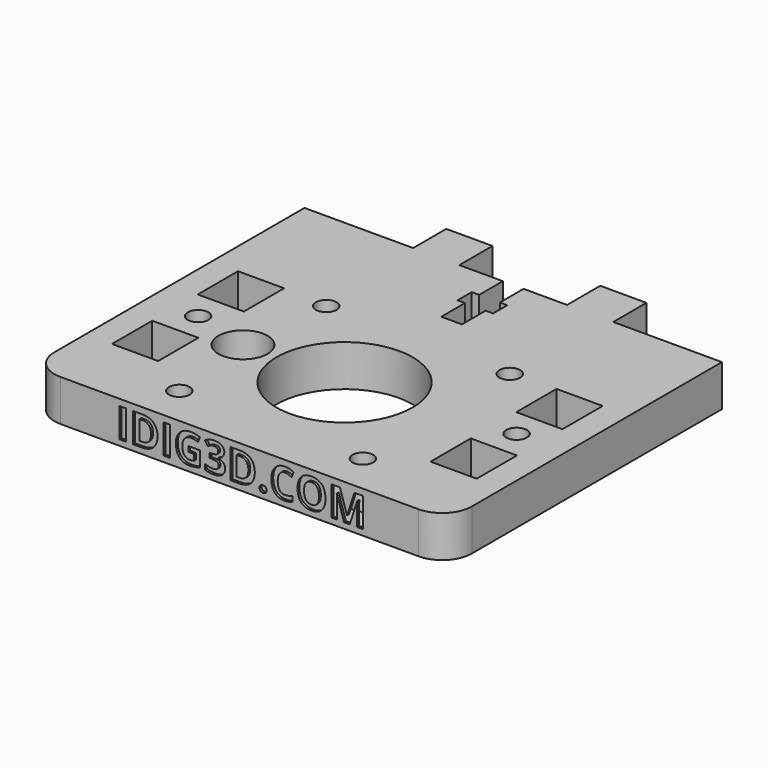
from build123d import *

# Parameters (mm, degrees)
F0_W         = 7.8
F0_H         = 7
F0_H_2       = 8.5
F0_R         = 1.75
F0_R_2       = 4.15
F0_R_3       = 11.5
F1_DEPTH     = 7
F2_TEXT_SIZE = 6.9444444444
F3_DEPTH     = 0.4


# Not quite as in the source:
# - Text() gives the source's letters only with a copy of the font that has no kerning and outlines rounded to 1/6400 em; it was checked with that copy


with BuildPart() as f1:
    # F0 (on Top) → F1 (new body)
    with BuildSketch(Plane.XY):
        with Locations((-13, 32.4)):
            Rectangle(F0_W, F0_H)
        with Locations((13, 32.4)):
            Rectangle(F0_W, F0_H)
        with BuildLine():
            Line((-16.9, 28.9), (-35.25, 28.9))
            Line((-35.25, 28.9), (-35.25, -23.9))
            ThreePointArc((-35.25, -23.9), (-33.7855339059, -27.4355339059), (-30.25, -28.9))
            Line((-30.25, -28.9), (30.25, -28.9))
            ThreePointArc((30.25, -28.9), (33.7855339059, -27.4355339059), (35.25, -23.9))
            Line((35.25, -23.9), (35.25, 28.9))
            Line((35.25, 28.9), (16.9, 28.9))
            Line((16.9, 28.9), (9.1, 28.9))
            Line((9.1, 28.9), (1.75, 28.9))
            Line((1.75, 28.9), (1.75, 23.9))
            Line((1.75, 23.9), (3, 23.9))
            Line((3, 23.9), (3, 20.9))
            Line((3, 20.9), (1.75, 20.9))
            Line((1.75, 20.9), (1.75, 15.9))
            Line((1.75, 15.9), (-1.75, 15.9))
            Line((-1.75, 15.9), (-1.75, 20.9))
            Line((-1.75, 20.9), (-3, 20.9))
            Line((-3, 20.9), (-3, 23.9))
            Line((-3, 23.9), (-1.75, 23.9))
            Line((-1.75, 23.9), (-1.75, 28.9))
            Line((-1.75, 28.9), (-9.1, 28.9))
            Line((-9.1, 28.9), (-16.9, 28.9))
        make_face()
        with Locations((-26.9, -13.05)):
            Rectangle(F0_W, F0_H_2, mode=Mode.SUBTRACT)
        with Locations((-15.5, -22.2)):
            Circle(F0_R, mode=Mode.SUBTRACT)
        with Locations((-26.9, -4)):
            Circle(F0_R, mode=Mode.SUBTRACT)
        with Locations((-17.15, -6.7)):
            Circle(F0_R_2, mode=Mode.SUBTRACT)
        with Locations((15.5, -22.2)):
            Circle(F0_R, mode=Mode.SUBTRACT)
        with Locations((26.9, -13.05)):
            Rectangle(F0_W, F0_H_2, mode=Mode.SUBTRACT)
        with Locations((0, -6.7)):
            Circle(F0_R_3, mode=Mode.SUBTRACT)
        with Locations((26.9, -4)):
            Circle(F0_R, mode=Mode.SUBTRACT)
        with Locations((-26.9, 5.05)):
            Rectangle(F0_W, F0_H_2, mode=Mode.SUBTRACT)
        with Locations((-15.5, 8.8)):
            Circle(F0_R, mode=Mode.SUBTRACT)
        with Locations((15.5, 8.8)):
            Circle(F0_R, mode=Mode.SUBTRACT)
        with Locations((26.9, 5.05)):
            Rectangle(F0_W, F0_H_2, mode=Mode.SUBTRACT)
    extrude(amount=F1_DEPTH)

    # F2 (on face) → F3 (cut)
    with BuildSketch(Plane.XZ.offset(28.9)):
        with Locations((-20.8642578125, 0.9745190581)):
            Text('IDIG3D.COM', F2_TEXT_SIZE, font='Open Sans', font_style=FontStyle.BOLD, text_align=(TextAlign.LEFT, TextAlign.BOTTOM))
    extrude(amount=-F3_DEPTH, mode=Mode.SUBTRACT)


solid = f1.part
